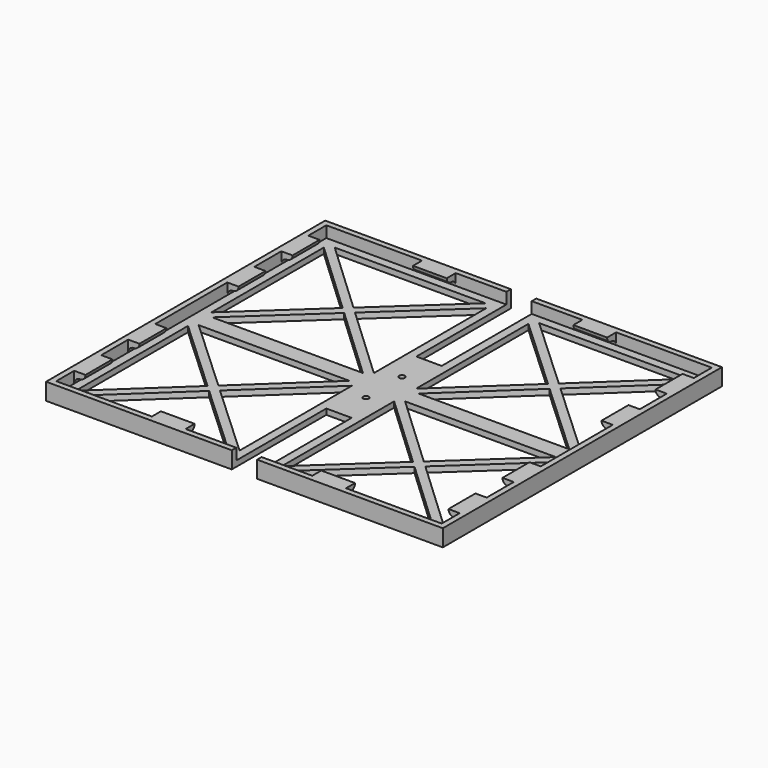
from build123d import *

# Parameters (mm, degrees)
F0_W     = 64
F0_H     = 120
F2_DEPTH = 2
F3_DEPTH = 6
F4_W     = 6
F4_H     = 12
F4_W_2   = 12
F4_H_2   = 6
F5_DEPTH = 2
F7_DEPTH = 2
F8_W     = 9
F8_H     = 40
F8_R     = 1
F9_DEPTH = 2
F10_R    = 1.99999
F11_R    = 1.99999


# Not quite as in the source:
# - a fillet or chamfer is up to 0.001 mm smaller than in the source, because OpenCascade refuses the exact size


with BuildPart() as f2:
    # F0 (on Top) → F2 (new body)
    with BuildSketch(Plane.XY):
        with Locations((-36.5, 0)):
            Rectangle(F0_W, F0_H)
    extrude(amount=F2_DEPTH)

    # F1 (on Top) → F3 (join)
    with BuildSketch(Plane.XY):
        Polygon((-4.5, 60), (-4.5, 62), (-70.5, 62), (-70.5, -62), (-4.5, -62), (-4.5, -60), (-68.5, -60), (-68.5, 60), align=None)
    extrude(amount=F3_DEPTH)

    # F4 (on face) → F5 (join)
    with BuildSketch(Plane.XY.offset(6)):
        with Locations((-67.5, 46)):
            Rectangle(F4_W, F4_H)
        with Locations((-28.5, 59)):
            Rectangle(F4_W_2, F4_H_2)
        with Locations((-67.5, 22)):
            Rectangle(F4_W, F4_H)
        with Locations((-28.5, -59)):
            Rectangle(F4_W_2, F4_H_2)
        with Locations((-67.5, -22)):
            Rectangle(F4_W, F4_H)
        with Locations((-67.5, -46)):
            Rectangle(F4_W, F4_H)
    extrude(amount=-F5_DEPTH)


with BuildPart() as f2b:
    # F0 (on Top) → F2, piece 2 (new body)
    with BuildSketch(Plane.XY):
        with Locations((36.5, 0)):
            Rectangle(F0_W, F0_H)
    extrude(amount=F2_DEPTH)

    # F1 (on Top) → F3, piece 2 (join)
    with BuildSketch(Plane.XY):
        Polygon((70.5, -62), (70.5, 62), (4.5, 62), (4.5, 60), (68.5, 60), (68.5, -60), (4.5, -60), (4.5, -62), align=None)
    extrude(amount=F3_DEPTH)

    # F4 (on face) → F5, piece 2 (join)
    with BuildSketch(Plane.XY.offset(6)):
        with Locations((67.5, 46)):
            Rectangle(F4_W, F4_H)
        with Locations((67.5, -22)):
            Rectangle(F4_W, F4_H)
        with Locations((67.5, -46)):
            Rectangle(F4_W, F4_H)
        with Locations((28.5, 59)):
            Rectangle(F4_W_2, F4_H_2)
        with Locations((67.5, 22)):
            Rectangle(F4_W, F4_H)
        with Locations((28.5, -59)):
            Rectangle(F4_W_2, F4_H_2)
    extrude(amount=-F5_DEPTH)


with BuildPart() as f7_tool:
    # F6 (on face) → F7 (new body)
    with BuildSketch(Plane(origin=(0, 0, 0), x_dir=(1, 0, 0), z_dir=(0, 0, -1))):
        Polygon((-9.5378331968, 57.0000003456), (-63.1068291486, 57.0000003456), (-36.4934644097, 32.0499709028), align=None)
        Polygon((-7.5, 4.8685980187), (-7.5, 54.7983564456), (-34.2993455202, 29.9929844439), align=None)
        Polygon((-9.8931712199, 3), (-36.5065294908, 27.9500233789), (-63.4621541524, 3), align=None)
        Polygon((-65.4999873492, 5.2016438999), (-38.7006483802, 30.0070098378), (-65.5, 55.1314019813), align=None)
        Polygon((-63.4621541524, -3), (-36.5065294908, -27.9500233789), (-9.8931712199, -3), align=None)
        Polygon((-7.5, -4.8685980187), (-34.2993455202, -29.9929844439), (-7.5, -54.7983564456), align=None)
        Polygon((-9.5378331968, -57.0000003456), (-36.4934644097, -32.0499709028), (-63.1068291486, -57.0000003456), align=None)
        Polygon((-65.5, -55.1314019813), (-38.7006483802, -30.0070098378), (-65.4999873492, -5.2016438999), align=None)
        Polygon((7.5, -54.7983564456), (34.2993455202, -29.9929844439), (7.5, -4.8685980187), align=None)
        Polygon((63.1068291486, -57.0000003456), (36.4934644097, -32.0499709028), (9.5378331968, -57.0000003456), align=None)
        Polygon((65.5, -55.1314019813), (65.4999873492, -5.2016438999), (38.7006483802, -30.0070098378), align=None)
        Polygon((36.5065294908, -27.9500233789), (63.4621541524, -3), (9.8931712199, -3), align=None)
        Polygon((63.4621541524, 3), (36.5065294908, 27.9500233789), (9.8931712199, 3), align=None)
        Polygon((7.5, 4.8685980187), (34.2993455202, 29.9929844439), (7.5, 54.7983564456), align=None)
        Polygon((9.5378331968, 57.0000003456), (36.4934644097, 32.0499709028), (63.1068291486, 57.0000003456), align=None)
        Polygon((65.5, 55.1314019813), (38.7006483802, 30.0070098378), (65.4999873492, 5.2016438999), align=None)
    extrude(amount=-F7_DEPTH)


with BuildPart() as f2_1:
    add(f2.part)

    # F7: cut by f7_tool
    add(f7_tool.part, mode=Mode.SUBTRACT)



with BuildPart() as f2b_1:
    add(f2b.part)

    # F7: cut by f7_tool
    add(f7_tool.part, mode=Mode.SUBTRACT)


with BuildPart() as f2_2:
    add(f2_1.part)

    add(f2b_1.part)  # F9 merges F2b
    # F8 (on face) → F9 (join)
    with BuildSketch(Plane(origin=(0, 0, 0), x_dir=(1, 0, 0), z_dir=(0, 0, -1))):
        Rectangle(F8_W, F8_H)
        with Locations((0, -8)):
            Circle(F8_R, mode=Mode.SUBTRACT)
        with Locations((0, 8)):
            Circle(F8_R, mode=Mode.SUBTRACT)
    extrude(amount=-F9_DEPTH)

    # F10 (radius 2 in the source; OpenCascade refuses exactly that, so slightly less here)
    f10_edges = [f2_2.edges().sort_by_distance(p)[0] for p in [
        (28.5, -56, 4),
        (-28.5, -56, 4),
        (64.5, -46, 4),
        (64.5, -22, 4),
        (-64.5, -46, 4),
        (-64.5, -22, 4),
        (64.5, 22, 4),
        (64.5, 46, 4),
        (-28.5, 56, 4),
        (28.5, 56, 4),
        (-64.5, 22, 4),
        (-64.5, 46, 4),
    ]]
    fillet(f10_edges, radius=F10_R)

    # F11 (radius 2 in the source; OpenCascade refuses exactly that, so slightly less here)
    f11_edges = [f2_2.edges().sort_by_distance(p)[0] for p in [
        (28.5, -60, 4),
        (-28.5, -60, 4),
        (-68.5, -46, 4),
        (-68.5, -22, 4),
        (68.5, -46, 4),
        (68.5, -22, 4),
        (68.5, 46, 4),
        (68.5, 22, 4),
        (28.5, 60, 4),
        (-28.5, 60, 4),
        (-68.5, 22, 4),
        (-68.5, 46, 4),
    ]]
    fillet(f11_edges, radius=F11_R)


solid = f2_2.part
